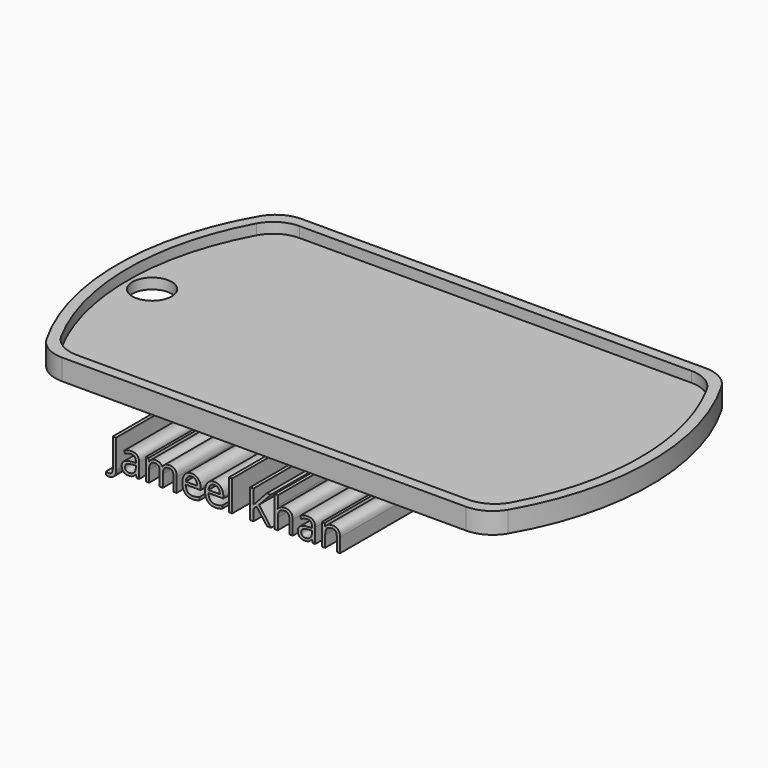
from build123d import *

# Parameters (mm, degrees)
F0_R         = 1.8739594118
F1_DEPTH     = 1
F3_DEPTH     = 1
F4_TEXT_SIZE = 3.8590314539
F5_DEPTH     = 25.4


# Not quite as in the source:
# - Text() gives the source's letters only with a copy of the font that has no kerning and outlines rounded to 1/6400 em; it was checked with that copy


with BuildPart() as f1:
    # F0 (on Top) → F1 (new body)
    with BuildSketch(Plane.XY):
        with BuildLine():
            ThreePointArc((-19.2474145991, 14.2875), (-20.8349145991, 13.862130657), (-21.9970452561, 12.7))
            ThreePointArc((-21.9970452561, 12.7), (-25.4, 0), (-21.9970452561, -12.7))
            ThreePointArc((-21.9970452561, -12.7), (-20.8349145991, -13.862130657), (-19.2474145991, -14.2875))
            Line((-19.2474145991, -14.2875), (19.2474145991, -14.2875))
            ThreePointArc((19.2474145991, -14.2875), (20.8349145991, -13.862130657), (21.9970452561, -12.7))
            ThreePointArc((21.9970452561, -12.7), (25.4, 0), (21.9970452561, 12.7))
            ThreePointArc((21.9970452561, 12.7), (20.8349145991, 13.862130657), (19.2474145991, 14.2875))
            Line((19.2474145991, 14.2875), (-19.2474145991, 14.2875))
        make_face()
        with Locations((-22.0978986472, 0)):
            Circle(F0_R, mode=Mode.SUBTRACT)
    extrude(amount=F1_DEPTH)

    # F2 (on face) → F3 (join)
    with BuildSketch(Plane.XY.offset(1)):
        with BuildLine():
            Line((19.2474145991, 14.2875), (-19.2474145991, 14.2875))
            ThreePointArc((-19.2474145991, 14.2875), (-20.8349145991, 13.862130657), (-21.9970452561, 12.7))
            ThreePointArc((-21.9970452561, 12.7), (-25.4, 0), (-21.9970452561, -12.7))
            ThreePointArc((-21.9970452561, -12.7), (-20.8349145991, -13.862130657), (-19.2474145991, -14.2875))
            Line((-19.2474145991, -14.2875), (19.2474145991, -14.2875))
            ThreePointArc((19.2474145991, -14.2875), (20.8349145991, -13.862130657), (21.9970452561, -12.7))
            ThreePointArc((21.9970452561, -12.7), (25.4, 0), (21.9970452561, 12.7))
            ThreePointArc((21.9970452561, 12.7), (20.8349145991, 13.862130657), (19.2474145991, 14.2875))
        make_face()
        with BuildLine():
            ThreePointArc((-21.4526124879, 11.6252061249), (-20.2856017842, 12.8404540819), (-18.6611352482, 13.2875))
            Line((-18.6611352482, 13.2875), (18.6611352482, 13.2875))
            ThreePointArc((18.6611352482, 13.2875), (20.2856017842, 12.8404540819), (21.4526124879, 11.6252061249))
            ThreePointArc((21.4526124879, 11.6252061249), (24.4, 0), (21.4526124879, -11.6252061249))
            ThreePointArc((21.4526124879, -11.6252061249), (20.2856017842, -12.8404540819), (18.6611352482, -13.2875))
            Line((18.6611352482, -13.2875), (-18.6611352482, -13.2875))
            ThreePointArc((-18.6611352482, -13.2875), (-20.2856017842, -12.8404540819), (-21.4526124879, -11.6252061249))
            ThreePointArc((-21.4526124879, -11.6252061249), (-24.4, 0), (-21.4526124879, 11.6252061249))
        make_face(mode=Mode.SUBTRACT)
    extrude(amount=F3_DEPTH)


with BuildPart() as f5:
    # F4 (on face) → F5 (new body)
    with BuildSketch(Plane.XZ.offset(-13.2875)):
        with Locations((-16.515006253, -7.2579295374)):
            Text('Jameel Khan', F4_TEXT_SIZE, font='Open Sans', text_align=(TextAlign.LEFT, TextAlign.BOTTOM))
    extrude(amount=F5_DEPTH)


solid = Compound([f1.part, f5.part])
